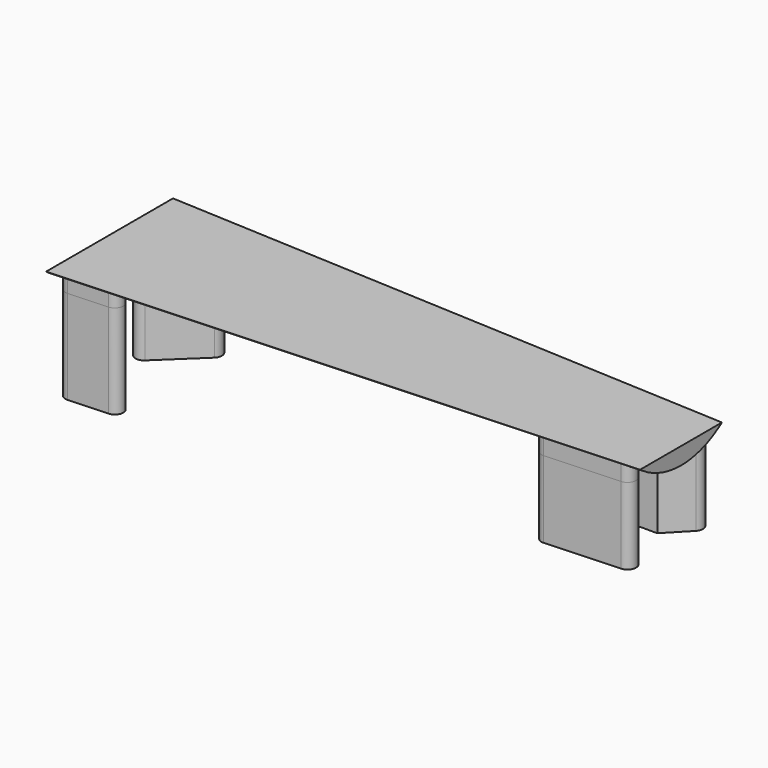
from build123d import *

# Parameters (mm, degrees)
F1_DEPTH     = 2
F3_DEPTH     = 13
F4_DEPTH     = 11
F5_R         = 1.5
F6_DEPTH     = 8
F7_T4_DEPTH  = 97.0812194284
F7_T9_DEPTH  = 97.0812194284
F7_T14_DEPTH = 97.0812194284
F7_T20_DEPTH = 97.0812194284
F7_T25_DEPTH = 97.0812194284
F7_T31_DEPTH = 97.0812194284
F8_R         = 1


# Not quite as in the source:
# - a fillet or chamfer that OpenCascade refuses, or shapes differently, is made with other operations: its cross-section is extruded or revolved along the edge and cut away or added


with BuildPart() as f1:
    # F0 (on Top) → F1 (new body)
    with BuildSketch(Plane.XY):
        Polygon((0, 9.3), (0, 0), (67, 0), (67, 6), align=None)
    extrude(amount=F1_DEPTH)

    # F2 (on face) → F3 (join)
    with BuildSketch(Plane.XY.offset(2)):
        Polygon((0.7854075007, 8.5), (0.7854075007, 0.5), (8.7757214003, 8.1064472258), align=None)
    extrude(amount=-F3_DEPTH)

    # F2 (on face) → F4 (join)
    with BuildSketch(Plane.XY.offset(2)):
        Polygon((62.9, 1.65), (66.9, 5.8), (53.9157399132, 6.439523258), (57.3, 1.65), align=None)
    extrude(amount=-F4_DEPTH)

    # F5 (on face) → F6 (cut)
    with BuildSketch(Plane(origin=(0, 0, -11), x_dir=(1, 0, 0), z_dir=(0, 0, -1))):
        with Locations((3.1854075007, -5.9788816921)):
            Circle(F5_R)
        with Locations((60.0157399132, -3.9364085902)):
            Circle(F5_R)
    extrude(amount=-F6_DEPTH, mode=Mode.SUBTRACT)

    # F7: fillet of radius 10 on 1 edges, made by hand


with BuildPart() as f7_tool2:
    # F7_s3 → F7_t4 (new body)
    with BuildSketch(Plane(origin=(81.5248873918, -4.0154049014, 0), x_dir=(0, 0, 1), z_dir=(-0.9987892374, 0.0491940968, 0))):
        with BuildLine():
            ThreePointArc((2, 9.2887399083), (0.5131670195, 6.4510175684), (0, 3.2887399083))
            Line((0, 3.2887399083), (0, 9.2887399083))
            Line((0, 9.2887399083), (2, 9.2887399083))
        make_face()
    extrude(amount=F7_T4_DEPTH)

    split(bisect_by=Plane(origin=(0.4468822571, 9.0730640082, 0), x_dir=(0, 0, 1), z_dir=(0.0491940968, 0.9987892374, 0)), keep=Keep.TOP)


with BuildPart() as f1_1:
    add(f1.part)

    # F7_t1: cut F7_tool2
    add(f7_tool2.part, mode=Mode.SUBTRACT)


with BuildPart() as f7_tool7:
    # F7_s8 → F7_t9 (new body)
    with BuildSketch(Plane(origin=(81.5248873918, -4.0154049014, 0), x_dir=(0, 0, 1), z_dir=(-0.9987892374, 0.0491940968, 0))):
        with BuildLine():
            ThreePointArc((2, 9.2887399083), (0.5131670195, 6.4510175684), (0, 3.2887399083))
            Line((0, 3.2887399083), (0, 9.2887399083))
            Line((0, 9.2887399083), (2, 9.2887399083))
        make_face()
    extrude(amount=F7_T9_DEPTH)

    split(bisect_by=Plane(origin=(31.7828354278, -30.6340582437, 0), x_dir=(0, 0, 1), z_dir=(0.7199990803, -0.6939750171, 0)), keep=Keep.TOP)


with BuildPart() as f1_2:
    add(f1_1.part)

    # F7_t6: cut F7_tool7
    add(f7_tool7.part, mode=Mode.SUBTRACT)


with BuildPart() as f7_tool12:
    # F7_s13 → F7_t14 (new body)
    with BuildSketch(Plane(origin=(81.5248873918, -4.0154049014, 0), x_dir=(0, 0, 1), z_dir=(-0.9987892374, 0.0491940968, 0))):
        with BuildLine():
            ThreePointArc((2, 9.2887399083), (0.5131670195, 6.4510175684), (0, 3.2887399083))
            Line((0, 3.2887399083), (0, 9.2887399083))
            Line((0, 9.2887399083), (2, 9.2887399083))
        make_face()
    extrude(amount=F7_T14_DEPTH)

    split(bisect_by=Plane(origin=(38.996012386, 27.554443554, 0), x_dir=(0, 0, 1), z_dir=(-0.816693011, -0.5770723748, 0)), keep=Keep.TOP)

    split(bisect_by=Plane(origin=(0.1236877347, -0.1299297552, 0), x_dir=(0, 0, 1), z_dir=(0.6894947075, -0.7242907209, 0)), keep=Keep.TOP)


with BuildPart() as f1_3:
    add(f1_2.part)

    # F7_t11: cut F7_tool12
    add(f7_tool12.part, mode=Mode.SUBTRACT)


with BuildPart() as f7_tool18:
    # F7_s19 → F7_t20 (new body)
    with BuildSketch(Plane(origin=(81.5248873918, -4.0154049014, 0), x_dir=(0, 0, 1), z_dir=(-0.9987892374, 0.0491940968, 0))):
        with BuildLine():
            ThreePointArc((2, 9.2887399083), (0.5131670195, 6.4510175684), (0, 3.2887399083))
            Line((0, 3.2887399083), (0, 9.2887399083))
            Line((0, 9.2887399083), (2, 9.2887399083))
        make_face()
    extrude(amount=F7_T20_DEPTH)

    split(bisect_by=Plane.XZ.offset(-1.65), keep=Keep.TOP)


with BuildPart() as f1_4:
    add(f1_3.part)

    # F7_t17: cut F7_tool18
    add(f7_tool18.part, mode=Mode.SUBTRACT)


with BuildPart() as f7_tool23:
    # F7_s24 → F7_t25 (new body)
    with BuildSketch(Plane(origin=(81.5248873918, -4.0154049014, 0), x_dir=(0, 0, 1), z_dir=(-0.9987892374, 0.0491940968, 0))):
        with BuildLine():
            ThreePointArc((2, 9.2887399083), (0.5131670195, 6.4510175684), (0, 3.2887399083))
            Line((0, 3.2887399083), (0, 9.2887399083))
            Line((0, 9.2887399083), (2, 9.2887399083))
        make_face()
    extrude(amount=F7_T25_DEPTH)

    split(bisect_by=Plane(origin=(0.419544275, 8.518020129, 0), x_dir=(0, 0, 1), z_dir=(0.0491940968, 0.9987892374, 0)), keep=Keep.TOP)

    split(bisect_by=Plane(origin=(0.1236877347, -0.1299297552, 0), x_dir=(0, 0, 1), z_dir=(-0.6894947075, 0.7242907209, 0)), keep=Keep.TOP)


with BuildPart() as f1_5:
    add(f1_4.part)

    # F7_t22: cut F7_tool23
    add(f7_tool23.part, mode=Mode.SUBTRACT)


with BuildPart() as f7_tool29:
    # F7_s30 → F7_t31 (new body)
    with BuildSketch(Plane(origin=(81.5248873918, -4.0154049014, 0), x_dir=(0, 0, 1), z_dir=(-0.9987892374, 0.0491940968, 0))):
        with BuildLine():
            ThreePointArc((2, 9.2887399083), (0.5131670195, 6.4510175684), (0, 3.2887399083))
            Line((0, 3.2887399083), (0, 9.2887399083))
            Line((0, 9.2887399083), (2, 9.2887399083))
        make_face()
    extrude(amount=F7_T31_DEPTH)

    split(bisect_by=Plane.YZ.offset(0.7854075007), keep=Keep.BOTTOM)


with BuildPart() as f1_6:
    add(f1_5.part)

    # F7_t28: cut F7_tool29
    add(f7_tool29.part, mode=Mode.SUBTRACT)

    # F8
    f8_edges = [f1_6.edges().sort_by_distance(p)[0] for p in [
        (0.785408, 8.5, -4.758713),
        (8.775721, 8.106447, -4.758713),
        (0.785408, 0.5, -5.5),
        (66.9, 5.8, -3.574746),
        (53.91574, 6.439523, -3.574746),
    ]]
    fillet(f8_edges, radius=F8_R)

    # F9: F1 across plane


with BuildPart() as f1_7:
    add(f1_6.part)
    add(f1_6.part.mirror(Plane.XZ))


solid = f1_7.part
